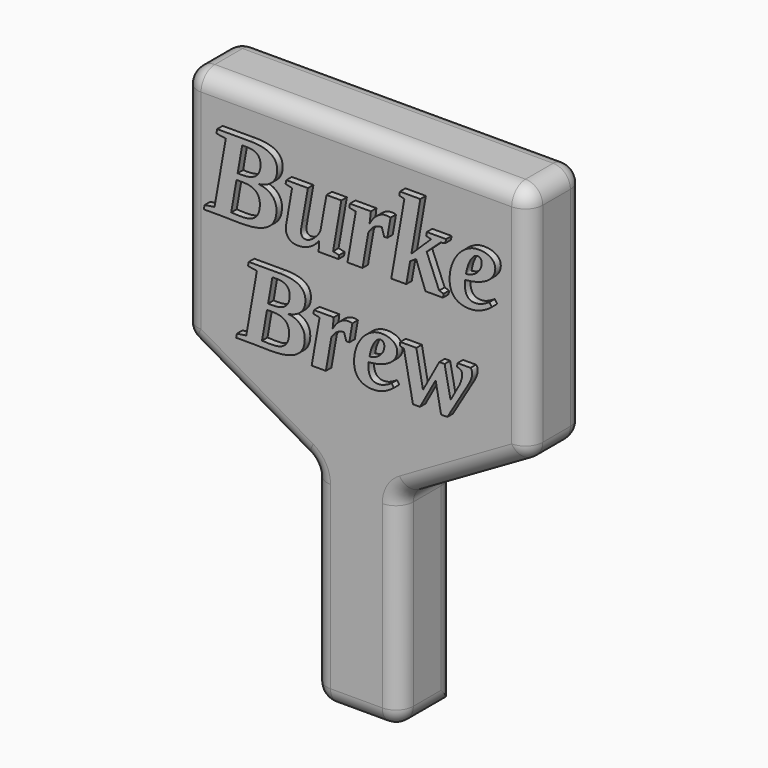
from build123d import *

# Parameters (mm, degrees)
F1_DEPTH     = 20
F2_R         = 5
F4_D         = 7.9375
F4_DEPTH     = 26
F4_TIP       = 2.3846655818
F5_TEXT_SIZE = 33.1889010138
F6_DEPTH     = 2
F7_TEXT_SIZE = 31.3595855712
F8_DEPTH     = 2


# Not quite as in the source:
# - Text() gives the source's letters only with a copy of the font that has no kerning and outlines rounded to 1/6400 em; it was checked with that copy


with BuildPart() as f1:
    # F0 (on Front) → F1 (new body)
    with BuildSketch(Plane.XZ):
        Polygon((50, 61.2133667238), (0, 61.2133667238), (-50, 61.2133667238), (-50, -7.1359981816), (-12.5, -28.7866332762), (-12.5, -88.7866332762), (0, -88.7866332762), (12.5, -88.7866332762), (12.5, -28.7866332762), (50, -7.1359981816), align=None)
    extrude(amount=F1_DEPTH)

    # F2
    f2_edges = [f1.edges().sort_by_distance(p)[0] for p in [
        (50, -10, -7.135998),
        (50, -10, 61.213367),
        (50, 0, 27.038684),
        (50, -20, 27.038684),
        (0, -20, 61.213367),
        (-50, -20, 27.038684),
        (-31.25, -20, -17.961316),
        (-12.5, -20, -58.786633),
        (0, -20, -88.786633),
        (12.5, -20, -58.786633),
        (31.25, -20, -17.961316),
        (-50, -10, 61.213367),
        (0, 0, 61.213367),
        (12.5, -10, -88.786633),
        (12.5, -10, -28.786633),
        (12.5, 0, -58.786633),
        (-12.5, -10, -28.786633),
        (-12.5, -10, -88.786633),
        (-12.5, 0, -58.786633),
        (-50, -10, -7.135998),
        (-50, 0, 27.038684),
        (-31.25, 0, -17.961316),
        (31.25, 0, -17.961316),
    ]]
    fillet(f2_edges, radius=F2_R)

    # F4
    with Locations(Plane(origin=(0, 0, -88.7866332762), x_dir=(1, 0, 0), z_dir=(0, 0, -1))):
        with Locations((0, 7.5)):
            Hole(F4_D / 2, depth=F4_DEPTH)
            with Locations((0, 0, -(F4_DEPTH + F4_TIP / 2))):  # 118° drill point
                Cone(0, F4_D / 2, F4_TIP, mode=Mode.SUBTRACT)

    # F5 (on face) → F6 (join)
    with BuildSketch(Plane.XZ.offset(20)):
        with Locations((-42.2697514296, 27.8832800686)):
            Text('Burke', F5_TEXT_SIZE, font='Tinos', font_style=FontStyle.BOLDITALIC, text_align=(TextAlign.LEFT, TextAlign.BOTTOM))
    extrude(amount=F6_DEPTH)

    # F7 (on face) → F8 (join)
    with BuildSketch(Plane.XZ.offset(20)):
        with Locations((-32.9275644035, -1.8150219694)):
            Text('Brew', F7_TEXT_SIZE, font='Tinos', font_style=FontStyle.BOLDITALIC, text_align=(TextAlign.LEFT, TextAlign.BOTTOM))
    extrude(amount=F8_DEPTH)


solid = f1.part
